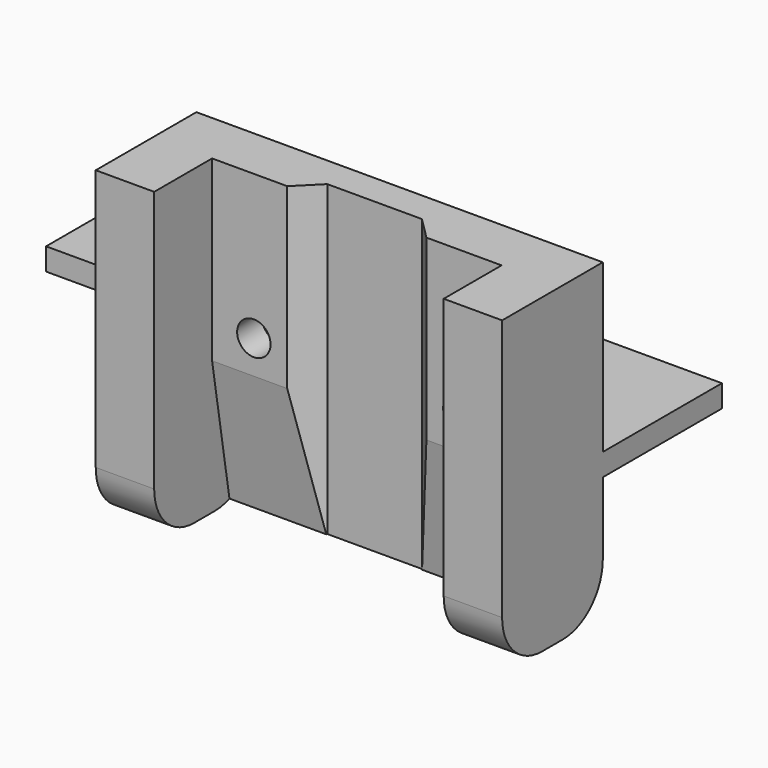
from build123d import *

# Parameters (mm, degrees)
F0_W           = 13.375
F0_H           = 2
F1_DEPTH       = 25
F2_R           = 1.75
F3_DEPTH       = 2
F4_W           = 11.3
F4_H           = 13
F5_DEPTH       = 25
F5_DEPTH_BACK  = 11.5
F6_W           = 26
F6_H           = 6.5
F7_DEPTH       = 13
F9_DEPTH       = 13
F11_DEPTH      = 19.75
F11_DEPTH_BACK = 6.25
F13_T1_DEPTH   = 27.75
F13_T3_DEPTH   = 27.75
F13_T5_DEPTH   = 59
F15_DEPTH      = 15
F16_W          = 5.5
F16_H          = 4.8968277758
F16_H_2        = 5.3132384717
F17_DEPTH      = 2
F18_DEPTH      = 2
F19_D          = 3


# Not quite as in the source:
# - a fillet or chamfer that OpenCascade refuses, or shapes differently, is made with other operations: its cross-section is extruded or revolved along the edge and cut away or added


with BuildPart() as f1:
    # F0 (on Right) → F1 (new body, symmetric)
    with BuildSketch(Plane.YZ):
        with Locations((6.6875, 1)):
            Rectangle(F0_W, F0_H)
    extrude(amount=F1_DEPTH, both=True)

    # F2 (on face) → F3 (cut, through all)
    with BuildSketch(Plane.XY.offset(2)):
        with Locations((-13, 4)):
            Circle(F2_R)
        with Locations((13, 4)):
            Circle(F2_R)
    extrude(amount=-F3_DEPTH, mode=Mode.SUBTRACT)

    # F4 (on Right) → F5 (join, two sides)
    with BuildSketch(Plane.YZ) as f5_sk:
        with Locations((-5.65, -4.5)):
            Rectangle(F4_W, F4_H)
    extrude(amount=F5_DEPTH)
    extrude(f5_sk.sketch, amount=-F5_DEPTH_BACK)

    # F6 (on face) → F7 (cut, through all)
    with BuildSketch(Plane(origin=(0, 0, -11), x_dir=(1, 0, 0), z_dir=(0, 0, -1))):
        with Locations((6.75, 8.05)):
            Rectangle(F6_W, F6_H)
    extrude(amount=-F7_DEPTH, mode=Mode.SUBTRACT)

    # F8 (on face) → F9 (cut, through all)
    with BuildSketch(Plane(origin=(0, 0, -11), x_dir=(1, 0, 0), z_dir=(0, 0, -1))):
        Polygon((13, 4.8), (0.5, 4.8), (2.5, 2.8), (11, 2.8), align=None)
    extrude(amount=-F9_DEPTH, mode=Mode.SUBTRACT)

    # F10 (on Right) → F11 (cut, two sides)
    with BuildSketch(Plane.YZ) as f11_sk:
        Polygon((-4.8, -11), (-2.8, -11), (-4.8, 1), align=None)
    extrude(amount=F11_DEPTH, mode=Mode.SUBTRACT)
    extrude(f11_sk.sketch, amount=-F11_DEPTH_BACK, mode=Mode.SUBTRACT)

    # F13: fillet of radius 4.5 on 3 edges, made by hand

    # F13_s2 → F13_t1 (cut)
    with BuildSketch(Plane.YZ.offset(-22.75)):
        with BuildLine():
            ThreePointArc((-6.8, -11), (-9.9819805153, -9.6819805153), (-11.3, -6.5))
            Line((-11.3, -6.5), (-11.3, -11))
            Line((-11.3, -11), (-6.8, -11))
        make_face()
    extrude(amount=F13_T1_DEPTH, mode=Mode.SUBTRACT)

    # F13_s4 → F13_t3 (cut)
    with BuildSketch(Plane.YZ.offset(8.5)):
        with BuildLine():
            ThreePointArc((-6.8, -11), (-9.9819805153, -9.6819805153), (-11.3, -6.5))
            Line((-11.3, -6.5), (-11.3, -11))
            Line((-11.3, -11), (-6.8, -11))
        make_face()
    extrude(amount=F13_T3_DEPTH, mode=Mode.SUBTRACT)

    # F13_s6 → F13_t5 (cut)
    with BuildSketch(Plane.YZ.offset(-22.75)):
        with BuildLine():
            ThreePointArc((0, -6.5), (-1.3180194847, -9.6819805153), (-4.5, -11))
            Line((-4.5, -11), (0, -11))
            Line((0, -11), (0, -6.5))
        make_face()
    extrude(amount=F13_T5_DEPTH, mode=Mode.SUBTRACT)

    # F14 (on face) → F15 (join)
    with BuildSketch(Plane.XY.offset(2)):
        Polygon((25, 0), (-11.5, 0), (-11.5, -11.3), (-6.25, -11.3), (-6.25, -4.8), (0.5, -4.8), (2.5, -2.8), (11, -2.8), (13, -4.8), (19.75, -4.8), (19.75, -11.3), (25, -11.3), align=None)
    extrude(amount=F15_DEPTH)

    # F16 (on face) → F17 (join)
    with BuildSketch(Plane(origin=(0, 0, 0), x_dir=(-1, 0, 0), z_dir=(0, 1, 0))):
        with Locations((-16.04918, 4.4484138879)):
            Rectangle(F16_W, F16_H)
        with Locations((2.45082, 4.6566192359)):
            Rectangle(F16_W, F16_H_2)
    extrude(amount=-F17_DEPTH)

    # F16 (on face) → F18 (cut)
    with BuildSketch(Plane(origin=(0, 0, 0), x_dir=(-1, 0, 0), z_dir=(0, 1, 0))):
        with Locations((-16.04918, 4.4484138879)):
            Rectangle(F16_W, F16_H)
        with Locations((2.45082, 4.6566192359)):
            Rectangle(F16_W, F16_H_2)
    extrude(amount=-F18_DEPTH, mode=Mode.SUBTRACT)

    # F19 (through all)
    with Locations(Plane.XZ.offset(4.8)):
        with Locations((16, 4), (-2.5, 4)):
            Hole(F19_D / 2)


solid = f1.part
